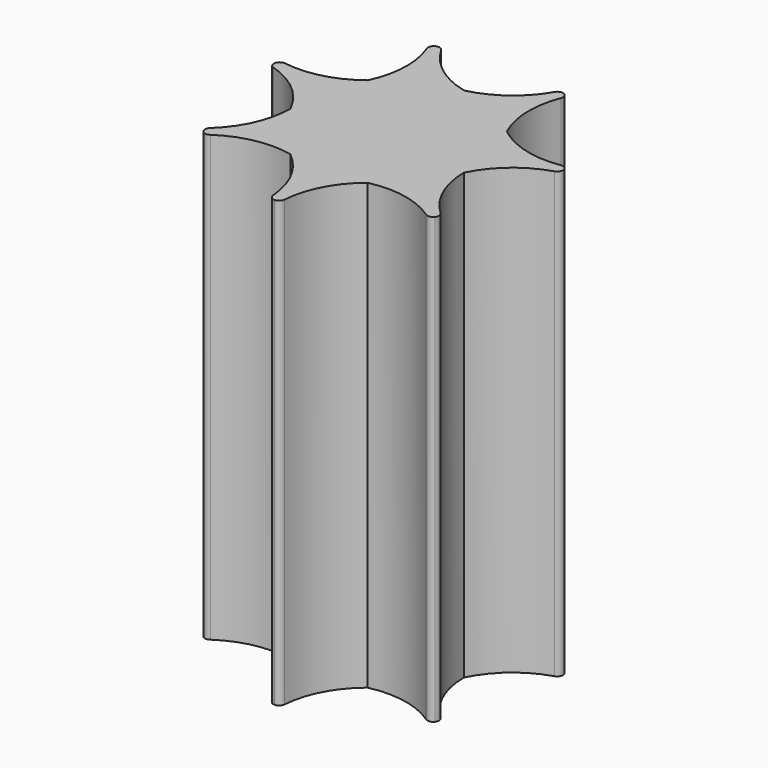
from build123d import *

# Parameters (mm, degrees)
F1_DEPTH    = 15
F2_T1_DEPTH = 15.9585845768


# Not quite as in the source:
# - a fillet or chamfer that OpenCascade refuses, or shapes differently, is made with other operations: its cross-section is extruded or revolved along the edge and cut away or added


with BuildPart() as f1:
    # F0 (on Top) → F1 (new body)
    with BuildSketch(Plane.XY):
        with BuildLine():
            ThreePointArc((2.9247837365, -0.6675628019), (3.7405193144, 0.3530547619), (4.9127228226, 0.9301368008))
            ThreePointArc((4.9127228226, 0.9301368008), (4.8746395609, 1.1126046698), (4.8297815528, 1.2935262471))
            ThreePointArc((4.8297815528, 1.2935262471), (3.5232761722, 1.3048591573), (2.3454944474, 1.8704694056))
            ThreePointArc((2.3454944474, 1.8704694056), (2.0561463183, 3.1445818043), (2.3358223454, 4.420852177))
            ThreePointArc((2.3358223454, 4.420852177), (2.1694186956, 4.5048443395), (2, 4.582575695))
            ThreePointArc((2, 4.582575695), (1.1765467932, 3.5681746103), (0, 3))
            ThreePointArc((0, 3), (-1.1765467932, 3.5681746103), (-2, 4.582575695))
            ThreePointArc((-2, 4.582575695), (-2.1694186956, 4.5048443395), (-2.3358223454, 4.420852177))
            ThreePointArc((-2.3358223454, 4.420852177), (-2.0561463183, 3.1445818043), (-2.3454944474, 1.8704694056))
            ThreePointArc((-2.3454944474, 1.8704694056), (-3.5232761722, 1.3048591573), (-4.8297815528, 1.2935262471))
            ThreePointArc((-4.8297815528, 1.2935262471), (-4.8746395609, 1.1126046698), (-4.9127228226, 0.9301368008))
            ThreePointArc((-4.9127228226, 0.9301368008), (-3.7405193144, 0.3530547619), (-2.9247837365, -0.6675628019))
            ThreePointArc((-2.9247837365, -0.6675628019), (-3.2169067319, -1.9410418555), (-4.0226390868, -2.9695748479))
            ThreePointArc((-4.0226390868, -2.9695748479), (-3.9091574123, -3.1174490093), (-3.7902428131, -3.2609905577))
            ThreePointArc((-3.7902428131, -3.2609905577), (-2.608204974, -2.7043297172), (-1.3016512174, -2.7029066037))
            ThreePointArc((-1.3016512174, -2.7029066037), (-0.4881409094, -3.725298761), (-0.1863673415, -4.9965255142))
            ThreePointArc((-0.1863673415, -4.9965255142), (0, -5), (0.1863673415, -4.9965255142))
            ThreePointArc((0.1863673415, -4.9965255142), (0.4881409094, -3.725298761), (1.3016512174, -2.7029066037))
            ThreePointArc((1.3016512174, -2.7029066037), (2.608204974, -2.7043297172), (3.7902428131, -3.2609905577))
            ThreePointArc((3.7902428131, -3.2609905577), (3.9091574123, -3.1174490093), (4.0226390868, -2.9695748479))
            ThreePointArc((4.0226390868, -2.9695748479), (3.2169067319, -1.9410418555), (2.9247837365, -0.6675628019))
        make_face()
    extrude(amount=F1_DEPTH)

    # F2: fillet of radius 0.2 on 14 edges, made by hand

    # F2_s2 → F2_t1 (cut)
    with BuildSketch(Plane.XY.offset(-0.4792922884)):
        with BuildLine():
            ThreePointArc((-3.9124710062, -3.1132893578), (-3.785825601, -3.1865171636), (-3.6432075854, -3.1539369268))
            ThreePointArc((-3.6432075854, -3.1539369268), (-3.7175366677, -3.2063492126), (-3.7902428131, -3.2609905577))
            ThreePointArc((-3.7902428131, -3.2609905577), (-3.8520648952, -3.1877258419), (-3.9124710062, -3.1132893578))
        make_face()
        with BuildLine():
            ThreePointArc((-3.8855510977, -2.8500477743), (-3.949049974, -2.9818402738), (-3.905839396, -3.121605134))
            ThreePointArc((-3.905839396, -3.121605134), (-3.9649679778, -3.0461498543), (-4.0226390868, -2.9695748479))
            ThreePointArc((-4.0226390868, -2.9695748479), (-3.9531890749, -2.9108504406), (-3.8855510977, -2.8500477743))
        make_face()
        with BuildLine():
            ThreePointArc((-0.1943444075, -4.814821897), (-0.1308957841, -4.946638597), (0.0053181385, -4.9999971717))
            ThreePointArc((0.0053181385, -4.9999971717), (-0.0905412424, -4.9991801611), (-0.1863673415, -4.9965255142))
            ThreePointArc((-0.1863673415, -4.9965255142), (-0.1889785578, -4.9056132393), (-0.1943444075, -4.814821897))
        make_face()
        with BuildLine():
            ThreePointArc((-0.0053181385, -4.9999971717), (0.1308957841, -4.946638597), (0.1943444075, -4.814821897))
            ThreePointArc((0.1943444075, -4.814821897), (0.1889785578, -4.9056132393), (0.1863673415, -4.9965255142))
            ThreePointArc((0.1863673415, -4.9965255142), (0.0905412424, -4.9991801611), (-0.0053181385, -4.9999971717))
        make_face()
        with BuildLine():
            ThreePointArc((3.6432075854, -3.1539369268), (3.785825601, -3.1865171636), (3.9124710062, -3.1132893578))
            ThreePointArc((3.9124710062, -3.1132893578), (3.8520648952, -3.1877258419), (3.7902428131, -3.2609905577))
            ThreePointArc((3.7902428131, -3.2609905577), (3.7175366677, -3.2063492126), (3.6432075854, -3.1539369268))
        make_face()
        with BuildLine():
            ThreePointArc((3.8855510977, -2.8500477743), (3.949049974, -2.9818402738), (3.905839396, -3.121605134))
            ThreePointArc((3.905839396, -3.121605134), (3.9649679778, -3.0461498543), (4.0226390868, -2.9695748479))
            ThreePointArc((4.0226390868, -2.9695748479), (3.9531890749, -2.9108504406), (3.8855510977, -2.8500477743))
        make_face()
        with BuildLine():
            ThreePointArc((4.7373499587, 0.8819268779), (4.8517430918, 0.973116687), (4.8734534064, 1.1177888421))
            ThreePointArc((4.8734534064, 1.1177888421), (4.8939875989, 1.024151054), (4.9127228226, 0.9301368008))
            ThreePointArc((4.9127228226, 0.9301368008), (4.8246709586, 0.9073611688), (4.7373499587, 0.8819268779))
        make_face()
        with BuildLine():
            ThreePointArc((4.8758202007, 1.1074192388), (4.7934889875, 1.228344594), (4.6508585605, 1.2608704528))
            ThreePointArc((4.6508585605, 1.2608704528), (4.7405675882, 1.2758421104), (4.8297815528, 1.2935262471))
            ThreePointArc((4.8297815528, 1.2935262471), (4.8536929553, 1.2006934229), (4.8758202007, 1.1074192388))
        make_face()
        with BuildLine():
            ThreePointArc((2.2641711887, 4.2536817555), (2.2641990769, 4.3999738244), (2.1646259913, 4.5071492451))
            ThreePointArc((2.1646259913, 4.5071492451), (2.2506378215, 4.4648213174), (2.3358223454, 4.420852177))
            ThreePointArc((2.3358223454, 4.420852177), (2.2987296122, 4.3378100833), (2.2641711887, 4.2536817555))
        make_face()
        with BuildLine():
            ThreePointArc((2.1742089456, 4.5025343375), (2.0283330241, 4.5135609289), (1.913974667, 4.4223275119))
            ThreePointArc((1.913974667, 4.4223275119), (1.9582020177, 4.5017995299), (2, 4.582575695))
            ThreePointArc((2, 4.582575695), (2.0874881401, 4.543390063), (2.1742089456, 4.5025343375))
        make_face()
        with BuildLine():
            ThreePointArc((-1.913974667, 4.4223275119), (-2.0283330241, 4.5135609289), (-2.1742089456, 4.5025343375))
            ThreePointArc((-2.1742089456, 4.5025343375), (-2.0874881401, 4.543390063), (-2, 4.582575695))
            ThreePointArc((-2, 4.582575695), (-1.9582020177, 4.5017995299), (-1.913974667, 4.4223275119))
        make_face()
        with BuildLine():
            ThreePointArc((-2.1646259913, 4.5071492451), (-2.2641990769, 4.3999738244), (-2.2641711887, 4.2536817555))
            ThreePointArc((-2.2641711887, 4.2536817555), (-2.2987296122, 4.3378100833), (-2.3358223454, 4.420852177))
            ThreePointArc((-2.3358223454, 4.420852177), (-2.2506378215, 4.4648213174), (-2.1646259913, 4.5071492451))
        make_face()
        with BuildLine():
            ThreePointArc((-4.8734534064, 1.1177888421), (-4.8517430918, 0.973116687), (-4.7373499587, 0.8819268779))
            ThreePointArc((-4.7373499587, 0.8819268779), (-4.8246709586, 0.9073611688), (-4.9127228226, 0.9301368008))
            ThreePointArc((-4.9127228226, 0.9301368008), (-4.8939875989, 1.024151054), (-4.8734534064, 1.1177888421))
        make_face()
        with BuildLine():
            ThreePointArc((-4.6508585605, 1.2608704528), (-4.7934889875, 1.228344594), (-4.8758202007, 1.1074192388))
            ThreePointArc((-4.8758202007, 1.1074192388), (-4.8536929553, 1.2006934229), (-4.8297815528, 1.2935262471))
            ThreePointArc((-4.8297815528, 1.2935262471), (-4.7405675882, 1.2758421104), (-4.6508585605, 1.2608704528))
        make_face()
    extrude(amount=F2_T1_DEPTH, mode=Mode.SUBTRACT)


solid = f1.part
